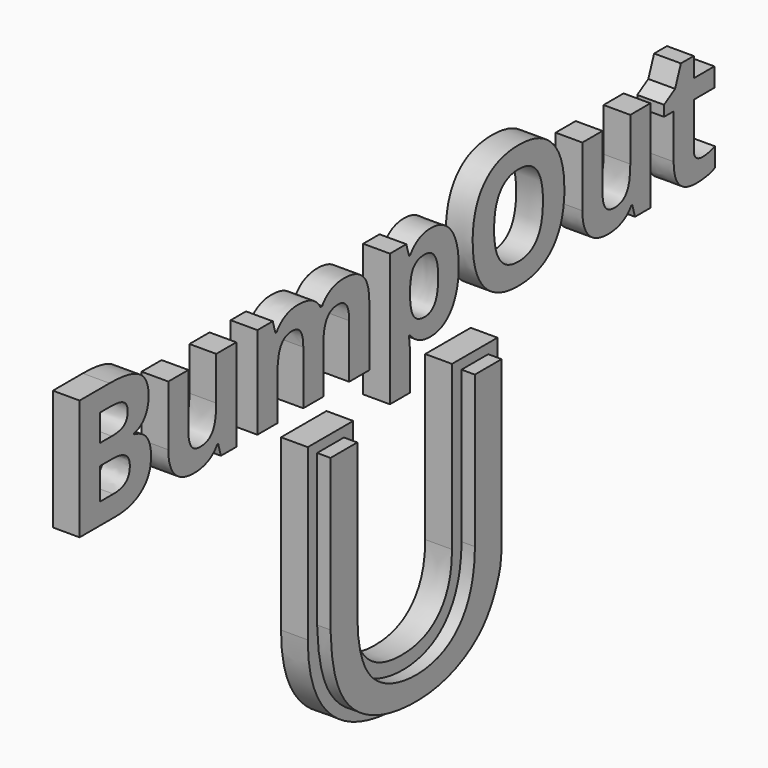
from build123d import *

# Parameters (mm, degrees)
F0_TEXT_SIZE = 160.0097140504
F1_DEPTH     = 25.4
F2_TEXT_SIZE = 374.1168520517
F3_DEPTH     = 25.4
F5_DEPTH     = 12.7


# Not quite as in the source:
# - Text() gives the source's letters only with a copy of the font that has no kerning and outlines rounded to 1/6400 em; it was checked with that copy


with BuildPart() as f1:
    # F0 (on Right) → F1 (new body)
    with BuildSketch(Plane.YZ):
        with Locations((-77.6318386197, -43.7022522092)):
            Text('BumpOut', F0_TEXT_SIZE, font='Open Sans', font_style=FontStyle.BOLD, text_align=(TextAlign.LEFT, TextAlign.BOTTOM))
    extrude(amount=F1_DEPTH)


with BuildPart() as f3:
    # F2 (on Right) → F3 (new body)
    with BuildSketch(Plane.YZ):
        with Locations((184.8020255566, -335.7262313366)):
            Text('U', F2_TEXT_SIZE, font='Arimo', font_style=FontStyle.BOLD, text_align=(TextAlign.LEFT, TextAlign.BOTTOM))
    extrude(amount=F3_DEPTH)


with BuildPart() as f5:
    # F4 (on face) → F5 (new body)
    with BuildSketch(Plane.YZ.offset(25.4)):
        with BuildLine():
            Line((250.072141179, -87.6952544172), (218.322141179, -87.6952544172))
            Line((218.322141179, -87.6952544172), (218.322141179, -231.3225850875))
            add(Edge.make_bspline(
                [(218.322141179, -231.3225850875), (219.1090066741, -256.3199820137), (226.4581602885, -295.6216808382), (268.1763465516, -327.7195530882), (320.6065744063, -334.704938157), (362.2048746464, -327.9831294809), (394.072219422, -309.7858355941), (409.6667155757, -288.6951300498), (419.6938524119, -264.2002021724), (421.3228225708, -251.6326904297), (421.1764400005, -231.3225850875)],
                knots=[0, 0, 0, 0, 0.158710634, 0.2958376015, 0.4386679259, 0.56772721, 0.6856779143, 0.7867634569, 0.8812463717, 1, 1, 1, 1], degree=3))
            Line((421.1764400005, -231.3225850875), (421.1764400005, -87.6952544172))
            Line((421.1764400005, -87.6952544172), (389.4264400005, -87.6952544172))
            Line((389.4264400005, -87.6952544172), (389.4264400005, -231.3225850875))
            add(Edge.make_bspline(
                [(250.072141179, -231.3225850875), (250.072141179, -251.734097405), (256.6711636932, -290.518118571), (301.1736743547, -312.6914797391), (351.0547861615, -309.445304483), (382.8511843472, -281.1108640537), (389.4264400005, -249.4984675103), (389.4264400005, -231.3225850875)],
                knots=[0, 0, 0, 0, 0.21903575, 0.4133910718, 0.6140950242, 0.795318123, 1, 1, 1, 1], degree=3))
            Line((250.072141179, -231.3225850875), (250.072141179, -87.6952544172))
        make_face()
    extrude(amount=F5_DEPTH)


solid = Compound([f1.part, f3.part, f5.part])
